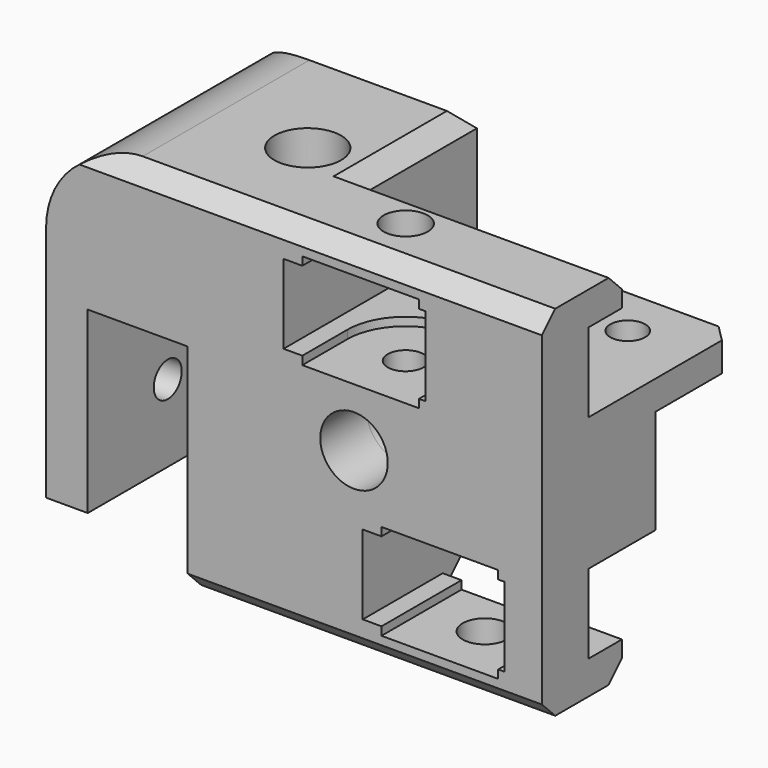
from build123d import *

# Parameters (mm, degrees)
F0_R           = 4.05
F1_DEPTH       = 7
F2_T1_DEPTH    = 63.387088135
F2_T3_DEPTH    = 52.7867319519
F4_DEPTH       = 22
F6_DEPTH       = 5
F7_R           = 4.05
F8_DEPTH       = 2
F9_R           = 4.05
F10_DEPTH      = 3
F11_R          = 4.05
F12_DEPTH      = 5
F13_T4_DEPTH   = 53.0035618315
F14_SIZE       = 2
F17_DEPTH      = 4
F15_R          = 4
F18_DEPTH      = 4.501
F18_DEPTH_BACK = 38.501
F19_R          = 2.3
F20_DEPTH      = 19.5
F21_R          = 2.65
F21_R_2        = 2.3
F22_DEPTH      = 3
F23_R          = 2.15
F24_DEPTH      = 22
F25_R          = 2.65
F25_R_2        = 2.15
F26_DEPTH      = 3
F28_DEPTH      = 1
F30_DEPTH      = 1
F31_R          = 2.1
F32_DEPTH      = 29.501
F33_T1_DEPTH   = 32.387088135
F33_T3_DEPTH   = 13.7849510361
F33_T8_DEPTH   = 29.2867319519
F34_R          = 2.1
F35_DEPTH      = 5


# Not quite as in the source:
# - a fillet or chamfer that OpenCascade refuses, or shapes differently, is made with other operations: its cross-section is extruded or revolved along the edge and cut away or added


with BuildPart() as f1:
    # F0 (on Front) → F1 (new body)
    with BuildSketch(Plane.XZ):
        with BuildLine():
            Line((0, 28.5), (0, 0))
            Line((0, 0), (5, 0))
            Line((5, 0), (5, 21.5))
            Line((5, 21.5), (17, 21.5))
            Line((17, 21.5), (17, -4.5))
            Line((17, -4.5), (59.5, -4.5))
            Line((59.5, -4.5), (59.5, 38.5))
            Line((59.5, 38.5), (10, 38.5))
            ThreePointArc((10, 38.5), (2.9289321881, 35.5710678119), (0, 28.5))
        make_face()
        Polygon((38, -0.5), (38, 9), (55, 9), (55, -0.5), (54.25, -0.5), (54.25, -1.5), (40.25, -1.5), (40.25, -0.5), align=None, mode=Mode.SUBTRACT)
        with Locations((36.95, 17)):
            Circle(F0_R, mode=Mode.SUBTRACT)
        Polygon((28.5, 25), (28.5, 34.5), (30.75, 34.5), (30.75, 35.5), (44.75, 35.5), (44.75, 34.5), (45.5, 34.5), (45.5, 25), align=None, mode=Mode.SUBTRACT)
    extrude(amount=F1_DEPTH)

    # F2: chamfer of 2 on 2 edges, made by hand

    # F2_s2 → F2_t1 (cut)
    with BuildSketch(Plane.YZ.offset(1.2562778409)):
        Polygon((-5, 38.5), (-7, 36.5), (-7, 38.5), align=None)
    extrude(amount=F2_T1_DEPTH, mode=Mode.SUBTRACT)

    # F2_s4 → F2_t3 (cut)
    with BuildSketch(Plane.YZ.offset(11.8566340241)):
        Polygon((-5, -4.5), (-7, -2.5), (-7, -4.5), align=None)
    extrude(amount=F2_T3_DEPTH, mode=Mode.SUBTRACT)

    # F3 (on face) → F4 (join)
    with BuildSketch(Plane(origin=(0, 0, 0), x_dir=(-1, 0, 0), z_dir=(0, 1, 0))):
        with BuildLine():
            Line((-59.5, 21.5), (-17, 21.5))
            Line((-17, 21.5), (-5, 21.5))
            Line((-5, 21.5), (-5, 0))
            Line((-5, 0), (0, 0))
            Line((0, 0), (0, 28.5))
            ThreePointArc((0, 28.5), (-2.9289321881, 35.5710678119), (-10, 38.5))
            Line((-10, 38.5), (-28.5, 38.5))
            Line((-28.5, 38.5), (-28.5, 34.5))
            Line((-28.5, 34.5), (-28.5, 25))
            Line((-28.5, 25), (-45.5, 25))
            Line((-45.5, 25), (-59.5, 25))
            Line((-59.5, 25), (-59.5, 21.5))
        make_face()
    extrude(amount=F4_DEPTH)

    # F5 (on face) → F6 (join)
    with BuildSketch(Plane(origin=(0, 0, 0), x_dir=(-1, 0, 0), z_dir=(0, 1, 0))):
        Polygon((-30.75, 34.5), (-28.5, 34.5), (-28.5, 38.5), (-59.5, 38.5), (-59.5, 34.5), (-45.5, 34.5), (-44.75, 34.5), (-44.75, 35.5), (-30.75, 35.5), align=None)
    extrude(amount=F6_DEPTH)

    # F7 (on face) → F8 (join)
    with BuildSketch(Plane(origin=(0, 0, 0), x_dir=(-1, 0, 0), z_dir=(0, 1, 0))):
        Polygon((-38, 9), (-38, -0.5), (-40.25, -0.5), (-40.25, -1.5), (-54.25, -1.5), (-54.25, -0.5), (-55, -0.5), (-59.5, -0.5), (-59.5, -4.5), (-17, -4.5), (-17, 21.5), (-59.5, 21.5), (-59.5, 9), (-55, 9), align=None)
        with Locations((-36.95, 17)):
            Circle(F7_R, mode=Mode.SUBTRACT)
    extrude(amount=F8_DEPTH)

    # F9 (on face) → F10 (join)
    with BuildSketch(Plane(origin=(0, 2, 0), x_dir=(-1, 0, 0), z_dir=(0, 1, 0))):
        Polygon((-21, -4.5), (-21, 21.5), (-59.5, 21.5), (-59.5, 9), (-38, 9), (-38, -0.5), (-40.25, -0.5), (-40.25, -1.5), (-54.25, -1.5), (-54.25, -0.5), (-59.5, -0.5), (-59.5, -4.5), align=None)
        with Locations((-36.95, 17)):
            Circle(F9_R, mode=Mode.SUBTRACT)
    extrude(amount=F10_DEPTH)

    # F11 (on face) → F12 (join)
    with BuildSketch(Plane(origin=(0, 5, 0), x_dir=(-1, 0, 0), z_dir=(0, 1, 0))):
        Polygon((-38, 9), (-38, -0.5), (-38, -4.5), (-21, -4.5), (-21, 21.5), (-59.5, 21.5), (-59.5, 9), align=None)
        with Locations((-36.95, 17)):
            Circle(F11_R, mode=Mode.SUBTRACT)
    extrude(amount=F12_DEPTH)

    # F13: chamfer of 7 on 1 edges, made by hand


with BuildPart() as f13_tool2:
    # F13_s3 → F13_t4 (new body)
    with BuildSketch(Plane.YZ.offset(56.0017809158)):
        Polygon((3, -4.5), (10, 2.5), (10, -4.5), align=None)
    extrude(amount=-F13_T4_DEPTH)

    split(bisect_by=Plane.YZ.offset(5), keep=Keep.TOP)


with BuildPart() as f1_1:
    add(f1.part)

    # F13_t1: cut F13_tool2
    add(f13_tool2.part, mode=Mode.SUBTRACT)

    # F14
    f14_edges = [f1_1.edges().sort_by_distance(p)[0] for p in [
        (44, 5, 38.5),
        (59.5, 22, 23.25),
    ]]
    chamfer(f14_edges, length=F14_SIZE)

    # F16 (on face) → F17 (cut)
    with BuildSketch(Plane(origin=(21, 0, 0), x_dir=(0, -1, 0), z_dir=(-1, 0, 0))):
        Polygon((-6, 21.5), (-10, 21.5), (-10, 2.5), (-6, -1.5), align=None)
    extrude(amount=-F17_DEPTH, mode=Mode.SUBTRACT)

    # F15 (on Top) → F18 (cut, two sides)
    with BuildSketch(Plane.XY) as f18_sk:
        with Locations((21, 6)):
            Circle(F15_R)
    extrude(amount=-F18_DEPTH, mode=Mode.SUBTRACT)
    extrude(f18_sk.sketch, amount=F18_DEPTH_BACK, mode=Mode.SUBTRACT)

    # F19 (on face) → F20 (cut)
    with BuildSketch(Plane(origin=(0, 0, -4.5), x_dir=(1, 0, 0), z_dir=(0, 0, -1))):
        with Locations((47.25, 0.25)):
            Circle(F19_R)
    extrude(amount=-F20_DEPTH, mode=Mode.SUBTRACT)

    # F21 (on face) → F22 (cut, through all)
    with BuildSketch(Plane(origin=(0, 0, -4.5), x_dir=(1, 0, 0), z_dir=(0, 0, -1))):
        with Locations((47.25, 0.25)):
            Circle(F21_R)
        with Locations((47.25, 0.25)):
            Circle(F21_R_2, mode=Mode.SUBTRACT)
    extrude(amount=-F22_DEPTH, mode=Mode.SUBTRACT)

    # F23 (on face) → F24 (cut)
    with BuildSketch(Plane.XY.offset(38.5)):
        with Locations((37.75, -0.25)):
            Circle(F23_R)
    extrude(amount=-F24_DEPTH, mode=Mode.SUBTRACT)

    # F25 (on face) → F26 (cut, through all)
    with BuildSketch(Plane.XY.offset(38.5)):
        with Locations((37.75, -0.25)):
            Circle(F25_R)
        with Locations((37.75, -0.25)):
            Circle(F25_R_2, mode=Mode.SUBTRACT)
    extrude(amount=-F26_DEPTH, mode=Mode.SUBTRACT)

    # F27 (on face) → F28 (cut)
    with BuildSketch(Plane.XY.offset(25)):
        with BuildLine():
            ThreePointArc((35.8959503782, -7), (32.1832079546, -4.4939163898), (30.75, -0.25))
            Line((30.75, -0.25), (30.75, -7))
            Line((30.75, -7), (35.8959503782, -7))
        make_face()
        with BuildLine():
            ThreePointArc((39.6040496218, -7), (43.3167920454, -4.4939163898), (44.75, -0.25))
            Line((44.75, -0.25), (39.9, -0.25))
            ThreePointArc((39.9, -0.25), (37.75, -2.4), (35.6, -0.25))
            Line((35.6, -0.25), (30.75, -0.25))
            ThreePointArc((30.75, -0.25), (32.1832079546, -4.4939163898), (35.8959503782, -7))
            Line((35.8959503782, -7), (39.6040496218, -7))
        make_face()
        with BuildLine():
            Line((39.9, -0.25), (44.75, -0.25))
            ThreePointArc((44.75, -0.25), (37.75, 6.75), (30.75, -0.25))
            Line((30.75, -0.25), (35.6, -0.25))
            ThreePointArc((35.6, -0.25), (37.75, 1.9), (39.9, -0.25))
        make_face()
        with BuildLine():
            Line((44.75, -7), (44.75, -0.25))
            ThreePointArc((44.75, -0.25), (43.3167920454, -4.4939163898), (39.6040496218, -7))
            Line((39.6040496218, -7), (44.75, -7))
        make_face()
    extrude(amount=-F28_DEPTH, mode=Mode.SUBTRACT)

    # F29 (on face) → F30 (cut)
    with BuildSketch(Plane(origin=(0, 0, 9), x_dir=(1, 0, 0), z_dir=(0, 0, -1))):
        with BuildLine():
            Line((44.95, 0.25), (40.25, 0.25))
            ThreePointArc((40.25, 0.25), (47.25, -6.75), (54.25, 0.25))
            Line((54.25, 0.25), (49.55, 0.25))
            ThreePointArc((49.55, 0.25), (47.25, -2.05), (44.95, 0.25))
        make_face()
        with BuildLine():
            ThreePointArc((45.3959503782, 7), (41.6832079546, 4.4939163898), (40.25, 0.25))
            Line((40.25, 0.25), (44.95, 0.25))
            ThreePointArc((44.95, 0.25), (47.25, 2.55), (49.55, 0.25))
            Line((49.55, 0.25), (54.25, 0.25))
            ThreePointArc((54.25, 0.25), (52.8167920454, 4.4939163898), (49.1040496218, 7))
            Line((49.1040496218, 7), (45.3959503782, 7))
        make_face()
        with BuildLine():
            Line((40.25, 7), (40.25, 0.25))
            ThreePointArc((40.25, 0.25), (41.6832079546, 4.4939163898), (45.3959503782, 7))
            Line((45.3959503782, 7), (40.25, 7))
        make_face()
        with BuildLine():
            ThreePointArc((49.1040496218, 7), (52.8167920454, 4.4939163898), (54.25, 0.25))
            Line((54.25, 0.25), (54.25, 7))
            Line((54.25, 7), (49.1040496218, 7))
        make_face()
    extrude(amount=-F30_DEPTH, mode=Mode.SUBTRACT)

    # F31 (on face) → F32 (cut, through all)
    with BuildSketch(Plane.XY.offset(25)):
        with Locations((36.9, 16)):
            Circle(F31_R)
        with Locations((51.4, 16)):
            Circle(F31_R)
    extrude(amount=-F32_DEPTH, mode=Mode.SUBTRACT)

    # F33: chamfer of 2 on 3 edges, made by hand

    # F33_s2 → F33_t1 (cut)
    with BuildSketch(Plane.YZ.offset(1.2562778409)):
        Polygon((22, 36.5), (20, 38.5), (22, 38.5), align=None)
    extrude(amount=F33_T1_DEPTH, mode=Mode.SUBTRACT)

    # F33_s4 → F33_t3 (cut)
    with BuildSketch(Plane.YZ.offset(50.8584149398)):
        Polygon((5, -2.5), (3, -4.5), (5, -4.5), align=None)
    extrude(amount=F33_T3_DEPTH, mode=Mode.SUBTRACT)


with BuildPart() as f33_tool6:
    # F33_s7 → F33_t8 (new body)
    with BuildSketch(Plane.XZ.offset(-27.1433659759)):
        Polygon((28.5, 36.5), (26.5, 38.5), (28.5, 38.5), align=None)
    extrude(amount=F33_T8_DEPTH)

    split(bisect_by=Plane(origin=(0, 20.75, 20.75), x_dir=(1, 0, 0), z_dir=(0, 0.7071067812, 0.7071067812)), keep=Keep.TOP)


with BuildPart() as f1_2:
    add(f1_1.part)

    # F33_t5: cut F33_tool6
    add(f33_tool6.part, mode=Mode.SUBTRACT)

    # F34 (on face) → F35 (cut, through all)
    with BuildSketch(Plane(origin=(0, 0, 0), x_dir=(0, -1, 0), z_dir=(-1, 0, 0))):
        with Locations((-5, 9.25)):
            Circle(F34_R)
    extrude(amount=-F35_DEPTH, mode=Mode.SUBTRACT)


solid = f1_2.part
